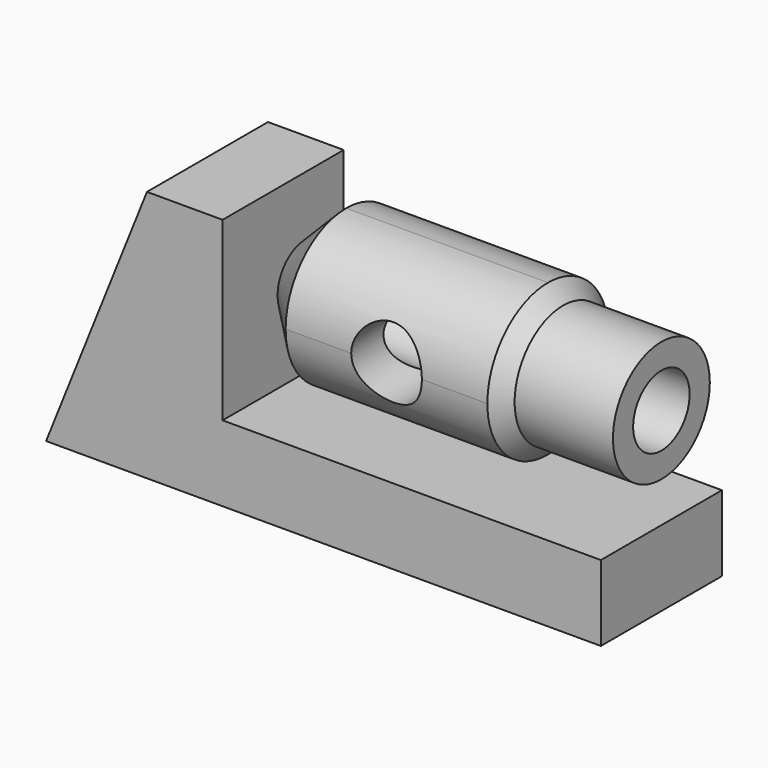
from build123d import *

# Parameters (mm, degrees)
F1_DEPTH = 6
F2_R     = 1.4
F3_DEPTH = 15
F5_R     = 1.4
F6_DEPTH = 25
F7_R     = 3
F7_R_2   = 2.4
F8_DEPTH = 4.5
F9_SIZE  = 0.59999


# Not quite as in the source:
# - a fillet or chamfer that OpenCascade refuses, or shapes differently, is made with other operations: its cross-section is extruded or revolved along the edge and cut away or added
# - a fillet or chamfer is up to 0.001 mm smaller than in the source, because OpenCascade refuses the exact size


with BuildPart() as f1:
    # F0 (on Front) → F1 (new body)
    with BuildSketch(Plane.XZ):
        Polygon((0, 4.5791433678), (-15, 4.5791433678), (-15, 11.5791433678), (-18, 11.5791433678), (-22, 1.5791433678), (0, 1.5791433678), align=None)
    extrude(amount=F1_DEPTH)


with BuildPart() as f3:
    # F2 (on face) → F3 (new body, through all)
    with BuildSketch(Plane.YZ.offset(-15)):
        with BuildLine():
            ThreePointArc((-6, 8.5791433678), (-3, 5.5791433678), (0, 8.5791433678))
            ThreePointArc((0, 8.5791433678), (-0.8786796564, 10.7004637114), (-3, 11.5791433678))
            ThreePointArc((-3, 11.5791433678), (-5.1213203436, 10.7004637114), (-6, 8.5791433678))
        make_face()
        with Locations((-3, 8.5791433678)):
            Circle(F2_R, mode=Mode.SUBTRACT)
    extrude(amount=F3_DEPTH)

    # F4: chamfer of 2.5 on 1 edges, made by hand

    # F4_s1 → F4_t2 (revolve, cut)
    with BuildSketch(Plane.XY.offset(8.5791433678)):
        Polygon((-12.5, 0), (-15, -2.5), (-15, 0), align=None)
    revolve(axis=Axis((-15, -3, 8.5791433678), (1, 0, 0)), mode=Mode.SUBTRACT)

    # F5 (on face) → F6 (cut)
    with BuildSketch(Plane.XZ.offset(6)):
        with Locations((-8.5, 8.5791433678)):
            Circle(F5_R)
    extrude(amount=-F6_DEPTH, mode=Mode.SUBTRACT)

    # F7 (on face) → F8 (cut)
    with BuildSketch(Plane.YZ):
        with Locations((-3, 8.5791433678)):
            Circle(F7_R)
        with Locations((-3, 8.5791433678)):
            Circle(F7_R_2, mode=Mode.SUBTRACT)
    extrude(amount=-F8_DEPTH, mode=Mode.SUBTRACT)

    # F9 (size 0.6 in the source; OpenCascade refuses exactly that, so slightly less here)
    f9_edges = [f3.edges().sort_by_distance(p)[0] for p in [
        (-4.5, -5.4, 8.579143),
    ]]
    chamfer(f9_edges, length=F9_SIZE)


solid = Compound([f1.part, f3.part])
